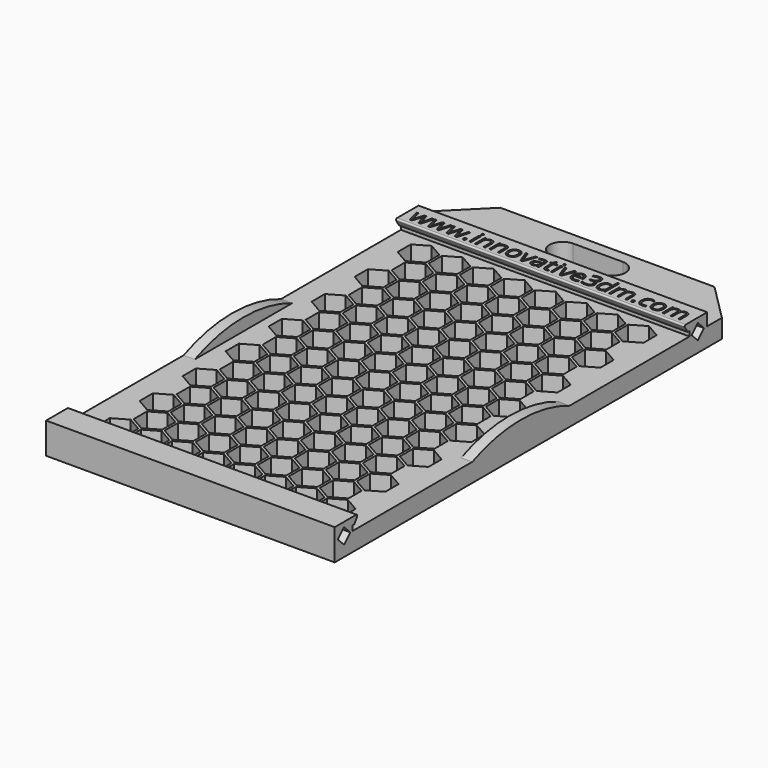
from build123d import *

# Parameters (mm, degrees)
F0_W         = 11.3907695115
F0_H         = 3.81
F1_DEPTH     = 29.5275
F3_DEPTH     = 2.286
F6_DEPTH     = 3.81
F7_TEXT_SIZE = 4.7833070588
F8_DEPTH     = 0.508
F10_DEPTH    = 3.81
F11_SIZE     = 7.62
F12_SIZE     = 7.62


# Not quite as in the source:
# - Text() gives the source's letters only with a copy of the font that has no kerning and outlines rounded to 1/6400 em; it was checked with that copy


with BuildPart() as f1:
    # F0 (on Right) → F1 (new body, symmetric)
    with BuildSketch(Plane.YZ):
        with BuildLine():
            Line((-47.625, 0), (0, 0))
            Line((0, 0), (47.625, 0))
            Line((47.625, 0), (47.625, 3.81))
            Line((47.625, 3.81), (47.625, 6.35))
            Line((47.625, 6.35), (42.1284169199, 6.35))
            ThreePointArc((42.1284169199, 6.35), (41.898214742, 6.2033450385), (41.9338416313, 5.9327319471))
            Line((41.9338416313, 5.9327319471), (42.6035709679, 4.826))
            Line((42.6035709679, 4.826), (42.8625, 4.826))
            Line((42.8625, 4.826), (43.113514781, 4.826))
            Line((43.113514781, 4.826), (43.113514781, 3.81))
            Line((43.113514781, 3.81), (42.8625, 3.81))
            Line((42.8625, 3.81), (0, 3.81))
            Line((0, 3.81), (-42.8625, 3.81))
            Line((-42.8625, 3.81), (-43.1086085737, 3.81))
            Line((-43.1086085737, 3.81), (-43.1086085737, 4.826))
            Line((-43.1086085737, 4.826), (-42.8625, 4.826))
            Line((-42.8625, 4.826), (-42.6015555859, 4.826))
            Line((-42.6015555859, 4.826), (-41.9338416313, 5.9327319471))
            ThreePointArc((-41.9338416313, 5.9327319471), (-41.898214742, 6.2033450385), (-42.1284169199, 6.35))
            Line((-42.1284169199, 6.35), (-47.625, 6.35))
            Line((-47.625, 6.35), (-47.625, 0))
        make_face()
        Polygon((-45.24375, 2.2225), (-46.83125, 3.81), (-45.24375, 5.3975), (-43.65625, 3.81), align=None, mode=Mode.SUBTRACT)
        Polygon((46.83125, 3.81), (45.24375, 2.2225), (43.65625, 3.81), (45.24375, 5.3975), align=None, mode=Mode.SUBTRACT)
        with Locations((53.3203847557, 1.905)):
            Rectangle(F0_W, F0_H)
    extrude(amount=F1_DEPTH, both=True)

    # F2 (on face) → F3 (join)
    with BuildSketch(Plane.YZ.offset(29.5275)):
        with BuildLine():
            Line((-12.4434078933, 3.81), (12.4434078933, 3.81))
            ThreePointArc((12.4434078933, 3.81), (0, 6.35), (-12.4434078933, 3.81))
        make_face()
    extrude(amount=-F3_DEPTH)

    # F4: F1 across plane


with BuildPart() as f1_1:
    add(f1.part)
    add(f1.part.mirror(Plane.YZ))

    # F5 (on face) → F6 (cut, through all)
    with BuildSketch(Plane.XY.offset(3.81)):
        Polygon((2.921, -1.6864401363), (2.921, 1.6864401363), (0, 3.3728802726), (-2.921, 1.6864401363), (-2.921, -1.6864401363), (0, -3.3728802726), align=None)
        Polygon((9.271, 1.6864401363), (6.35, 3.3728802726), (3.429, 1.6864401363), (3.429, -1.6864401363), (6.35, -3.3728802726), (9.271, -1.6864401363), align=None)
        Polygon((15.621, 1.6864401363), (12.7, 3.3728802726), (9.779, 1.6864401363), (9.779, -1.6864401363), (12.7, -3.3728802726), (15.621, -1.6864401363), align=None)
        Polygon((21.971, 1.6864401363), (19.05, 3.3728802726), (16.129, 1.6864401363), (16.129, -1.6864401363), (19.05, -3.3728802726), (21.971, -1.6864401363), align=None)
        Polygon((0.254, 3.8128211777), (3.175, 2.1263810414), (6.096, 3.8128211777), (6.096, 7.1857014503), (3.175, 8.8721415866), (0.254, 7.1857014503), align=None)
        Polygon((9.525, 8.8721415866), (6.604, 7.1857014503), (6.604, 3.8128211777), (9.525, 2.1263810414), (12.446, 3.8128211777), (12.446, 7.1857014503), align=None)
        Polygon((15.875, 8.8721415866), (12.954, 7.1857014503), (12.954, 3.8128211777), (15.875, 2.1263810414), (18.796, 3.8128211777), (18.796, 7.1857014503), align=None)
        Polygon((22.225, 8.8721415866), (19.304, 7.1857014503), (19.304, 3.8128211777), (22.225, 2.1263810414), (25.146, 3.8128211777), (25.146, 7.1857014503), align=None)
        Polygon((-9.271, 1.6864401363), (-9.271, -1.6864401363), (-6.35, -3.3728802726), (-3.429, -1.6864401363), (-3.429, 1.6864401363), (-6.35, 3.3728802726), align=None)
        Polygon((-15.621, 1.6864401363), (-15.621, -1.6864401363), (-12.7, -3.3728802726), (-9.779, -1.6864401363), (-9.779, 1.6864401363), (-12.7, 3.3728802726), align=None)
        Polygon((-21.971, 1.6864401363), (-21.971, -1.6864401363), (-19.05, -3.3728802726), (-16.129, -1.6864401363), (-16.129, 1.6864401363), (-19.05, 3.3728802726), align=None)
        Polygon((-6.096, 7.1857014503), (-6.096, 3.8128211777), (-3.175, 2.1263810414), (-0.254, 3.8128211777), (-0.254, 7.1857014503), (-3.175, 8.8721415866), align=None)
        Polygon((-12.446, 7.1857014503), (-12.446, 3.8128211777), (-9.525, 2.1263810414), (-6.604, 3.8128211777), (-6.604, 7.1857014503), (-9.525, 8.8721415866), align=None)
        Polygon((-18.796, 7.1857014503), (-18.796, 3.8128211777), (-15.875, 2.1263810414), (-12.954, 3.8128211777), (-12.954, 7.1857014503), (-15.875, 8.8721415866), align=None)
        Polygon((-25.146, 7.1857014503), (-25.146, 3.8128211777), (-22.225, 2.1263810414), (-19.304, 3.8128211777), (-19.304, 7.1857014503), (-22.225, 8.8721415866), align=None)
        Polygon((-9.779, 9.3120900637), (-9.779, 12.6849703363), (-12.7, 14.3714104726), (-15.621, 12.6849703363), (-15.621, 9.3120900637), (-12.7, 7.6256499274), align=None)
        Polygon((-12.446, 18.1842316503), (-12.446, 14.8113513777), (-9.525, 13.1249112414), (-6.604, 14.8113513777), (-6.604, 18.1842316503), (-9.525, 19.8706717866), align=None)
        Polygon((-19.05, 14.3714104726), (-21.971, 12.6849703363), (-21.971, 9.3120900637), (-19.05, 7.6256499274), (-16.129, 9.3120900637), (-16.129, 12.6849703363), align=None)
        Polygon((16.129, 9.3120900637), (19.05, 7.6256499274), (21.971, 9.3120900637), (21.971, 12.6849703363), (19.05, 14.3714104726), (16.129, 12.6849703363), align=None)
        Polygon((9.271, 9.3120900637), (9.271, 12.6849703363), (6.35, 14.3714104726), (3.429, 12.6849703363), (3.429, 9.3120900637), (6.35, 7.6256499274), align=None)
        Polygon((9.779, 9.3120900637), (12.7, 7.6256499274), (15.621, 9.3120900637), (15.621, 12.6849703363), (12.7, 14.3714104726), (9.779, 12.6849703363), align=None)
        Polygon((9.525, 19.8706717866), (6.604, 18.1842316503), (6.604, 14.8113513777), (9.525, 13.1249112414), (12.446, 14.8113513777), (12.446, 18.1842316503), align=None)
        Polygon((-9.271, 12.6849703363), (-9.271, 9.3120900637), (-6.35, 7.6256499274), (-3.429, 9.3120900637), (-3.429, 12.6849703363), (-6.35, 14.3714104726), align=None)
        Polygon((-15.875, 19.8706717866), (-18.796, 18.1842316503), (-18.796, 14.8113513777), (-15.875, 13.1249112414), (-12.954, 14.8113513777), (-12.954, 18.1842316503), align=None)
        Polygon((25.146, 18.1842316503), (22.225, 19.8706717866), (19.304, 18.1842316503), (19.304, 14.8113513777), (22.225, 13.1249112414), (25.146, 14.8113513777), align=None)
        Polygon((2.921, 12.6849703363), (0, 14.3714104726), (-2.921, 12.6849703363), (-2.921, 9.3120900637), (0, 7.6256499274), (2.921, 9.3120900637), align=None)
        Polygon((-3.175, 13.1249112414), (-0.254, 14.8113513777), (-0.254, 18.1842316503), (-3.175, 19.8706717866), (-6.096, 18.1842316503), (-6.096, 14.8113513777), align=None)
        Polygon((-22.225, 19.8706717866), (-25.146, 18.1842316503), (-25.146, 14.8113513777), (-22.225, 13.1249112414), (-19.304, 14.8113513777), (-19.304, 18.1842316503), align=None)
        Polygon((15.875, 13.1249112414), (18.796, 14.8113513777), (18.796, 18.1842316503), (15.875, 19.8706717866), (12.954, 18.1842316503), (12.954, 14.8113513777), align=None)
        Polygon((3.175, 13.1249112414), (6.096, 14.8113513777), (6.096, 18.1842316503), (3.175, 19.8706717866), (0.254, 18.1842316503), (0.254, 14.8113513777), align=None)
        Polygon((-9.779, 20.3106202637), (-9.779, 23.6835005363), (-12.7, 25.3699406726), (-15.621, 23.6835005363), (-15.621, 20.3106202637), (-12.7, 18.6241801274), align=None)
        Polygon((-12.446, 29.1827618503), (-12.446, 25.8098815777), (-9.525, 24.1234414414), (-6.604, 25.8098815777), (-6.604, 29.1827618503), (-9.525, 30.8692019866), align=None)
        Polygon((-19.05, 25.3699406726), (-21.971, 23.6835005363), (-21.971, 20.3106202637), (-19.05, 18.6241801274), (-16.129, 20.3106202637), (-16.129, 23.6835005363), align=None)
        Polygon((16.129, 20.3106202637), (19.05, 18.6241801274), (21.971, 20.3106202637), (21.971, 23.6835005363), (19.05, 25.3699406726), (16.129, 23.6835005363), align=None)
        Polygon((9.271, 20.3106202637), (9.271, 23.6835005363), (6.35, 25.3699406726), (3.429, 23.6835005363), (3.429, 20.3106202637), (6.35, 18.6241801274), align=None)
        Polygon((9.779, 20.3106202637), (12.7, 18.6241801274), (15.621, 20.3106202637), (15.621, 23.6835005363), (12.7, 25.3699406726), (9.779, 23.6835005363), align=None)
        Polygon((9.525, 30.8692019866), (6.604, 29.1827618503), (6.604, 25.8098815777), (9.525, 24.1234414414), (12.446, 25.8098815777), (12.446, 29.1827618503), align=None)
        Polygon((-9.271, 23.6835005363), (-9.271, 20.3106202637), (-6.35, 18.6241801274), (-3.429, 20.3106202637), (-3.429, 23.6835005363), (-6.35, 25.3699406726), align=None)
        Polygon((-15.875, 30.8692019866), (-18.796, 29.1827618503), (-18.796, 25.8098815777), (-15.875, 24.1234414414), (-12.954, 25.8098815777), (-12.954, 29.1827618503), align=None)
        Polygon((25.146, 29.1827618503), (22.225, 30.8692019866), (19.304, 29.1827618503), (19.304, 25.8098815777), (22.225, 24.1234414414), (25.146, 25.8098815777), align=None)
        Polygon((2.921, 23.6835005363), (0, 25.3699406726), (-2.921, 23.6835005363), (-2.921, 20.3106202637), (0, 18.6241801274), (2.921, 20.3106202637), align=None)
        Polygon((-3.175, 24.1234414414), (-0.254, 25.8098815777), (-0.254, 29.1827618503), (-3.175, 30.8692019866), (-6.096, 29.1827618503), (-6.096, 25.8098815777), align=None)
        Polygon((-22.225, 30.8692019866), (-25.146, 29.1827618503), (-25.146, 25.8098815777), (-22.225, 24.1234414414), (-19.304, 25.8098815777), (-19.304, 29.1827618503), align=None)
        Polygon((15.875, 24.1234414414), (18.796, 25.8098815777), (18.796, 29.1827618503), (15.875, 30.8692019866), (12.954, 29.1827618503), (12.954, 25.8098815777), align=None)
        Polygon((3.175, 24.1234414414), (6.096, 25.8098815777), (6.096, 29.1827618503), (3.175, 30.8692019866), (0.254, 29.1827618503), (0.254, 25.8098815777), align=None)
        Polygon((-9.779, 31.3091504637), (-9.779, 34.6820307363), (-12.7, 36.3684708726), (-15.621, 34.6820307363), (-15.621, 31.3091504637), (-12.7, 29.6227103274), align=None)
        Polygon((-12.446, 40.1812920503), (-12.446, 36.8084117777), (-9.525, 35.1219716414), (-6.604, 36.8084117777), (-6.604, 40.1812920503), (-9.525, 41.8677321866), align=None)
        Polygon((-19.05, 36.3684708726), (-21.971, 34.6820307363), (-21.971, 31.3091504637), (-19.05, 29.6227103274), (-16.129, 31.3091504637), (-16.129, 34.6820307363), align=None)
        Polygon((16.129, 31.3091504637), (19.05, 29.6227103274), (21.971, 31.3091504637), (21.971, 34.6820307363), (19.05, 36.3684708726), (16.129, 34.6820307363), align=None)
        Polygon((9.271, 31.3091504637), (9.271, 34.6820307363), (6.35, 36.3684708726), (3.429, 34.6820307363), (3.429, 31.3091504637), (6.35, 29.6227103274), align=None)
        Polygon((9.779, 31.3091504637), (12.7, 29.6227103274), (15.621, 31.3091504637), (15.621, 34.6820307363), (12.7, 36.3684708726), (9.779, 34.6820307363), align=None)
        Polygon((9.525, 41.8677321866), (6.604, 40.1812920503), (6.604, 36.8084117777), (9.525, 35.1219716414), (12.446, 36.8084117777), (12.446, 40.1812920503), align=None)
        Polygon((-9.271, 34.6820307363), (-9.271, 31.3091504637), (-6.35, 29.6227103274), (-3.429, 31.3091504637), (-3.429, 34.6820307363), (-6.35, 36.3684708726), align=None)
        Polygon((-15.875, 41.8677321866), (-18.796, 40.1812920503), (-18.796, 36.8084117777), (-15.875, 35.1219716414), (-12.954, 36.8084117777), (-12.954, 40.1812920503), align=None)
        Polygon((25.146, 40.1812920503), (22.225, 41.8677321866), (19.304, 40.1812920503), (19.304, 36.8084117777), (22.225, 35.1219716414), (25.146, 36.8084117777), align=None)
        Polygon((2.921, 34.6820307363), (0, 36.3684708726), (-2.921, 34.6820307363), (-2.921, 31.3091504637), (0, 29.6227103274), (2.921, 31.3091504637), align=None)
        Polygon((-3.175, 35.1219716414), (-0.254, 36.8084117777), (-0.254, 40.1812920503), (-3.175, 41.8677321866), (-6.096, 40.1812920503), (-6.096, 36.8084117777), align=None)
        Polygon((-22.225, 41.8677321866), (-25.146, 40.1812920503), (-25.146, 36.8084117777), (-22.225, 35.1219716414), (-19.304, 36.8084117777), (-19.304, 40.1812920503), align=None)
        Polygon((15.875, 35.1219716414), (18.796, 36.8084117777), (18.796, 40.1812920503), (15.875, 41.8677321866), (12.954, 40.1812920503), (12.954, 36.8084117777), align=None)
        Polygon((3.175, 35.1219716414), (6.096, 36.8084117777), (6.096, 40.1812920503), (3.175, 41.8677321866), (0.254, 40.1812920503), (0.254, 36.8084117777), align=None)
        Polygon((-3.175, -8.8721491586), (-0.254, -7.1857090223), (-0.254, -3.8128287497), (-3.175, -2.1263886134), (-6.096, -3.8128287497), (-6.096, -7.1857090223), align=None)
        Polygon((18.796, -7.1857090223), (18.796, -3.8128287497), (15.875, -2.1263886134), (12.954, -3.8128287497), (12.954, -7.1857090223), (15.875, -8.8721491586), align=None)
        Polygon((-18.796, -7.1857090223), (-15.875, -8.8721491586), (-12.954, -7.1857090223), (-12.954, -3.8128287497), (-15.875, -2.1263886134), (-18.796, -3.8128287497), align=None)
        Polygon((-19.304, -7.1857090223), (-19.304, -3.8128287497), (-22.225, -2.1263886134), (-25.146, -3.8128287497), (-25.146, -7.1857090223), (-22.225, -8.8721491586), align=None)
        Polygon((-6.35, -14.3714104726), (-3.429, -12.6849703363), (-3.429, -9.3120900637), (-6.35, -7.6256499274), (-9.271, -9.3120900637), (-9.271, -12.6849703363), align=None)
        Polygon((-12.7, -7.6256499274), (-15.621, -9.3120900637), (-15.621, -12.6849703363), (-12.7, -14.3714104726), (-9.779, -12.6849703363), (-9.779, -9.3120900637), align=None)
        Polygon((9.779, -12.6849703363), (12.7, -14.3714104726), (15.621, -12.6849703363), (15.621, -9.3120900637), (12.7, -7.6256499274), (9.779, -9.3120900637), align=None)
        Polygon((-12.446, -3.8128287497), (-12.446, -7.1857090223), (-9.525, -8.8721491586), (-6.604, -7.1857090223), (-6.604, -3.8128287497), (-9.525, -2.1263886134), align=None)
        Polygon((0.254, -3.8128287497), (0.254, -7.1857090223), (3.175, -8.8721491586), (6.096, -7.1857090223), (6.096, -3.8128287497), (3.175, -2.1263886134), align=None)
        Polygon((21.971, -9.3120900637), (19.05, -7.6256499274), (16.129, -9.3120900637), (16.129, -12.6849703363), (19.05, -14.3714104726), (21.971, -12.6849703363), align=None)
        Polygon((25.146, -7.1857090223), (25.146, -3.8128287497), (22.225, -2.1263886134), (19.304, -3.8128287497), (19.304, -7.1857090223), (22.225, -8.8721491586), align=None)
        Polygon((-19.05, -7.6256499274), (-21.971, -9.3120900637), (-21.971, -12.6849703363), (-19.05, -14.3714104726), (-16.129, -12.6849703363), (-16.129, -9.3120900637), align=None)
        Polygon((12.446, -7.1857090223), (12.446, -3.8128287497), (9.525, -2.1263886134), (6.604, -3.8128287497), (6.604, -7.1857090223), (9.525, -8.8721491586), align=None)
        Polygon((3.429, -12.6849703363), (6.35, -14.3714104726), (9.271, -12.6849703363), (9.271, -9.3120900637), (6.35, -7.6256499274), (3.429, -9.3120900637), align=None)
        Polygon((2.921, -12.6849703363), (2.921, -9.3120900637), (0, -7.6256499274), (-2.921, -9.3120900637), (-2.921, -12.6849703363), (0, -14.3714104726), align=None)
        Polygon((-3.175, -19.8706793586), (-0.254, -18.1842392223), (-0.254, -14.8113589497), (-3.175, -13.1249188134), (-6.096, -14.8113589497), (-6.096, -18.1842392223), align=None)
        Polygon((18.796, -18.1842392223), (18.796, -14.8113589497), (15.875, -13.1249188134), (12.954, -14.8113589497), (12.954, -18.1842392223), (15.875, -19.8706793586), align=None)
        Polygon((-18.796, -18.1842392223), (-15.875, -19.8706793586), (-12.954, -18.1842392223), (-12.954, -14.8113589497), (-15.875, -13.1249188134), (-18.796, -14.8113589497), align=None)
        Polygon((-19.304, -18.1842392223), (-19.304, -14.8113589497), (-22.225, -13.1249188134), (-25.146, -14.8113589497), (-25.146, -18.1842392223), (-22.225, -19.8706793586), align=None)
        Polygon((-6.35, -25.3699406726), (-3.429, -23.6835005363), (-3.429, -20.3106202637), (-6.35, -18.6241801274), (-9.271, -20.3106202637), (-9.271, -23.6835005363), align=None)
        Polygon((-12.7, -18.6241801274), (-15.621, -20.3106202637), (-15.621, -23.6835005363), (-12.7, -25.3699406726), (-9.779, -23.6835005363), (-9.779, -20.3106202637), align=None)
        Polygon((9.779, -23.6835005363), (12.7, -25.3699406726), (15.621, -23.6835005363), (15.621, -20.3106202637), (12.7, -18.6241801274), (9.779, -20.3106202637), align=None)
        Polygon((-12.446, -14.8113589497), (-12.446, -18.1842392223), (-9.525, -19.8706793586), (-6.604, -18.1842392223), (-6.604, -14.8113589497), (-9.525, -13.1249188134), align=None)
        Polygon((0.254, -14.8113589497), (0.254, -18.1842392223), (3.175, -19.8706793586), (6.096, -18.1842392223), (6.096, -14.8113589497), (3.175, -13.1249188134), align=None)
        Polygon((21.971, -20.3106202637), (19.05, -18.6241801274), (16.129, -20.3106202637), (16.129, -23.6835005363), (19.05, -25.3699406726), (21.971, -23.6835005363), align=None)
        Polygon((25.146, -18.1842392223), (25.146, -14.8113589497), (22.225, -13.1249188134), (19.304, -14.8113589497), (19.304, -18.1842392223), (22.225, -19.8706793586), align=None)
        Polygon((-19.05, -18.6241801274), (-21.971, -20.3106202637), (-21.971, -23.6835005363), (-19.05, -25.3699406726), (-16.129, -23.6835005363), (-16.129, -20.3106202637), align=None)
        Polygon((12.446, -18.1842392223), (12.446, -14.8113589497), (9.525, -13.1249188134), (6.604, -14.8113589497), (6.604, -18.1842392223), (9.525, -19.8706793586), align=None)
        Polygon((3.429, -23.6835005363), (6.35, -25.3699406726), (9.271, -23.6835005363), (9.271, -20.3106202637), (6.35, -18.6241801274), (3.429, -20.3106202637), align=None)
        Polygon((2.921, -23.6835005363), (2.921, -20.3106202637), (0, -18.6241801274), (-2.921, -20.3106202637), (-2.921, -23.6835005363), (0, -25.3699406726), align=None)
        Polygon((-3.175, -30.8692095586), (-0.254, -29.1827694223), (-0.254, -25.8098891497), (-3.175, -24.1234490134), (-6.096, -25.8098891497), (-6.096, -29.1827694223), align=None)
        Polygon((18.796, -29.1827694223), (18.796, -25.8098891497), (15.875, -24.1234490134), (12.954, -25.8098891497), (12.954, -29.1827694223), (15.875, -30.8692095586), align=None)
        Polygon((-18.796, -29.1827694223), (-15.875, -30.8692095586), (-12.954, -29.1827694223), (-12.954, -25.8098891497), (-15.875, -24.1234490134), (-18.796, -25.8098891497), align=None)
        Polygon((-19.304, -29.1827694223), (-19.304, -25.8098891497), (-22.225, -24.1234490134), (-25.146, -25.8098891497), (-25.146, -29.1827694223), (-22.225, -30.8692095586), align=None)
        Polygon((-6.35, -36.3684708726), (-3.429, -34.6820307363), (-3.429, -31.3091504637), (-6.35, -29.6227103274), (-9.271, -31.3091504637), (-9.271, -34.6820307363), align=None)
        Polygon((-12.7, -29.6227103274), (-15.621, -31.3091504637), (-15.621, -34.6820307363), (-12.7, -36.3684708726), (-9.779, -34.6820307363), (-9.779, -31.3091504637), align=None)
        Polygon((9.779, -34.6820307363), (12.7, -36.3684708726), (15.621, -34.6820307363), (15.621, -31.3091504637), (12.7, -29.6227103274), (9.779, -31.3091504637), align=None)
        Polygon((-12.446, -25.8098891497), (-12.446, -29.1827694223), (-9.525, -30.8692095586), (-6.604, -29.1827694223), (-6.604, -25.8098891497), (-9.525, -24.1234490134), align=None)
        Polygon((0.254, -25.8098891497), (0.254, -29.1827694223), (3.175, -30.8692095586), (6.096, -29.1827694223), (6.096, -25.8098891497), (3.175, -24.1234490134), align=None)
        Polygon((21.971, -31.3091504637), (19.05, -29.6227103274), (16.129, -31.3091504637), (16.129, -34.6820307363), (19.05, -36.3684708726), (21.971, -34.6820307363), align=None)
        Polygon((25.146, -29.1827694223), (25.146, -25.8098891497), (22.225, -24.1234490134), (19.304, -25.8098891497), (19.304, -29.1827694223), (22.225, -30.8692095586), align=None)
        Polygon((-19.05, -29.6227103274), (-21.971, -31.3091504637), (-21.971, -34.6820307363), (-19.05, -36.3684708726), (-16.129, -34.6820307363), (-16.129, -31.3091504637), align=None)
        Polygon((12.446, -29.1827694223), (12.446, -25.8098891497), (9.525, -24.1234490134), (6.604, -25.8098891497), (6.604, -29.1827694223), (9.525, -30.8692095586), align=None)
        Polygon((3.429, -34.6820307363), (6.35, -36.3684708726), (9.271, -34.6820307363), (9.271, -31.3091504637), (6.35, -29.6227103274), (3.429, -31.3091504637), align=None)
        Polygon((2.921, -34.6820307363), (2.921, -31.3091504637), (0, -29.6227103274), (-2.921, -31.3091504637), (-2.921, -34.6820307363), (0, -36.3684708726), align=None)
        Polygon((-19.304, -40.1812996223), (-19.304, -36.8084193497), (-22.225, -35.1219792134), (-25.146, -36.8084193497), (-25.146, -40.1812996223), (-22.225, -41.8677397586), align=None)
        Polygon((-15.875, -35.1219792134), (-18.796, -36.8084193497), (-18.796, -40.1812996223), (-15.875, -41.8677397586), (-12.954, -40.1812996223), (-12.954, -36.8084193497), align=None)
        Polygon((-9.525, -35.1219792134), (-12.446, -36.8084193497), (-12.446, -40.1812996223), (-9.525, -41.8677397586), (-6.604, -40.1812996223), (-6.604, -36.8084193497), align=None)
        Polygon((-6.096, -36.8084193497), (-6.096, -40.1812996223), (-3.175, -41.8677397586), (-0.254, -40.1812996223), (-0.254, -36.8084193497), (-3.175, -35.1219792134), align=None)
        Polygon((3.175, -35.1219792134), (0.254, -36.8084193497), (0.254, -40.1812996223), (3.175, -41.8677397586), (6.096, -40.1812996223), (6.096, -36.8084193497), align=None)
        Polygon((6.604, -36.8084193497), (6.604, -40.1812996223), (9.525, -41.8677397586), (12.446, -40.1812996223), (12.446, -36.8084193497), (9.525, -35.1219792134), align=None)
        Polygon((12.954, -36.8084193497), (12.954, -40.1812996223), (15.875, -41.8677397586), (18.796, -40.1812996223), (18.796, -36.8084193497), (15.875, -35.1219792134), align=None)
        Polygon((19.304, -36.8084193497), (19.304, -40.1812996223), (22.225, -41.8677397586), (25.146, -40.1812996223), (25.146, -36.8084193497), (22.225, -35.1219792134), align=None)
    extrude(amount=-F6_DEPTH, mode=Mode.SUBTRACT)

    # F7 (on face) → F8 (cut)
    with BuildSketch(Plane.XY.offset(6.35)):
        with Locations((-28.3166281879, 42.9656878114)):
            Text('www.innovative3dm.com', F7_TEXT_SIZE, font='Open Sans', text_align=(TextAlign.LEFT, TextAlign.BOTTOM))
    extrude(amount=-F8_DEPTH, mode=Mode.SUBTRACT)

    # F9 (on face) → F10 (cut, through all)
    with BuildSketch(Plane.XY.offset(3.81)):
        with BuildLine():
            Line((0, 51.2608849317), (5.08, 51.2608849317))
            ThreePointArc((5.08, 51.2608849317), (7.7548845797, 53.9357695115), (5.08, 56.6106540912))
            Line((5.08, 56.6106540912), (0, 56.6106540912))
            Line((0, 56.6106540912), (-5.08, 56.6106540912))
            ThreePointArc((-5.08, 56.6106540912), (-7.7548845797, 53.9357695115), (-5.08, 51.2608849317))
            Line((-5.08, 51.2608849317), (0, 51.2608849317))
        make_face()
    extrude(amount=-F10_DEPTH, mode=Mode.SUBTRACT)

    # F11
    f11_edges = [f1_1.edges().sort_by_distance(p)[0] for p in [
        (-29.5275, 59.01577, 1.905),
    ]]
    chamfer(f11_edges, length=F11_SIZE)

    # F12
    f12_edges = [f1_1.edges().sort_by_distance(p)[0] for p in [
        (29.5275, 59.01577, 1.905),
    ]]
    chamfer(f12_edges, length=F12_SIZE)


solid = f1_1.part
